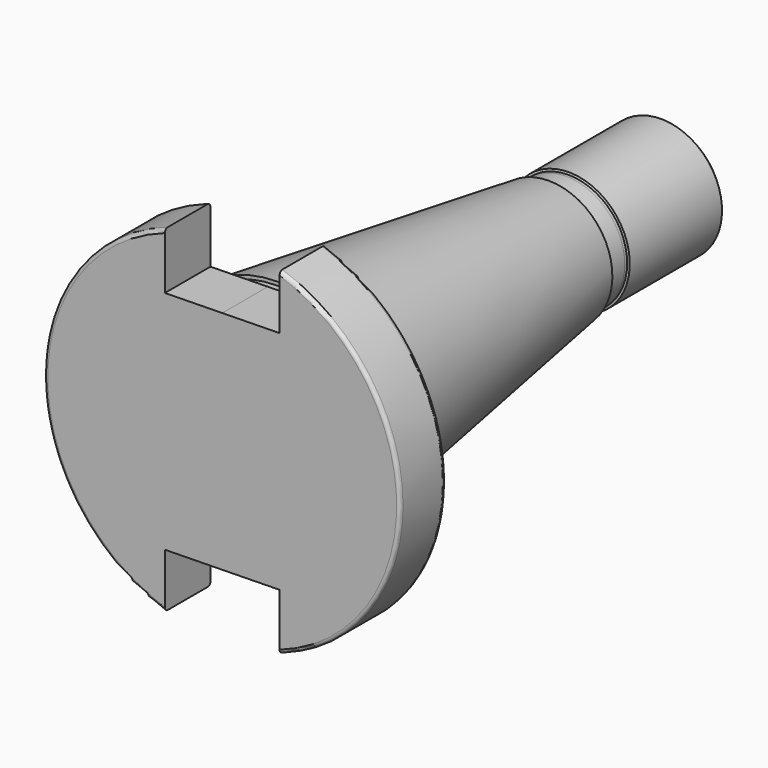
from build123d import *

# Parameters (mm, degrees)
F2_R             = 8.25
F3_DEPTH         = 3
F4_R             = 8.55
F5_DEPTH         = 17.2
F7_S5_R          = 8.25
F7_T6_DEPTH      = 14
F6_R             = 6.25
F8_DEPTH         = 4
F10_D            = 10.3
F10_DEPTH        = 25
F10_TIP          = 3.094432188
F11_R            = 0.5
F12_SIZE         = 0.5
F14_DEPTH        = 8
F14_COPIES_COUNT = 2


# Not quite as in the source:
# - a fillet or chamfer that OpenCascade refuses, or shapes differently, is made with other operations: its cross-section is extruded or revolved along the edge and cut away or added
# - a pattern or mirror of a feature is missing from the dataset's text; its kind, count and spacing are read off the source's solid


with BuildPart() as f1:
    # F0 (on Right) → F1 (revolve)
    with BuildSketch(Plane.YZ):
        Polygon((0, 25), (0, 0), (57.36, 0), (57.36, 8.9099957178), (9.6, 15.875), (9.6, 15.375), (8, 15.375), (8, 15.875), (8, 25), align=None)
    revolve(axis=Axis((0, 28.68, 0), (0, 1, 0)))

    # F2 (on face) → F3 (join)
    with BuildSketch(Plane(origin=(0, 57.36, 0), x_dir=(-1, 0, 0), z_dir=(0, 1, 0))):
        Circle(F2_R)
    extrude(amount=F3_DEPTH)

    # F4 (on face) → F5 (join)
    with BuildSketch(Plane(origin=(0, 60.36, 0), x_dir=(-1, 0, 0), z_dir=(0, 1, 0))):
        Circle(F4_R)
    extrude(amount=F5_DEPTH)

    # F7: chamfer of 0.5 x 1.8660254038 on 1 edges, made by hand


with BuildPart() as f7_tool2:
    # F7_s3 → F7_t4 (revolve)
    with BuildSketch(Plane.XY):
        Polygon((-8.55, 60.86), (-6.6839745962, 60.36), (-8.55, 60.36), align=None)
    revolve(axis=Axis((0, 60.36, 0), (0, 1, 0)))

    # F7_s5 → F7_t6 (cut, symmetric)
    with BuildSketch(Plane.XZ.offset(-60.6)):
        Circle(F7_S5_R)
    extrude(amount=F7_T6_DEPTH, both=True, mode=Mode.SUBTRACT)


with BuildPart() as f1_1:
    add(f1.part)

    # F7_t1: cut F7_tool2
    add(f7_tool2.part, mode=Mode.SUBTRACT)

    # F6 (on face) → F8 (cut)
    with BuildSketch(Plane(origin=(0, 77.56, 0), x_dir=(-1, 0, 0), z_dir=(0, 1, 0))):
        Circle(F6_R)
    extrude(amount=-F8_DEPTH, mode=Mode.SUBTRACT)

    # F10
    with Locations(Plane(origin=(0, 73.56, 0), x_dir=(-1, 0, 0), z_dir=(0, 1, 0))):
        with Locations((0, 0)):
            Hole(F10_D / 2, depth=F10_DEPTH)
            with Locations((0, 0, -(F10_DEPTH + F10_TIP / 2))):  # 118° drill point
                Cone(0, F10_D / 2, F10_TIP, mode=Mode.SUBTRACT)

    # F11
    f11_edges = [f1_1.edges().sort_by_distance(p)[0] for p in [
        (0, 8, -25),
        (0, 0, -25),
        (0, 4, 25),
    ]]
    fillet(f11_edges, radius=F11_R)

    # F12
    f12_edges = [f1_1.edges().sort_by_distance(p)[0] for p in [
        (8.55, 77.56, 0),
        (6.25, 77.56, 0),
        (5.15, 73.56, 0),
    ]]
    chamfer(f12_edges, length=F12_SIZE)

    # F13 (on face) → F14 (cut, through all)
    with BuildSketch(Plane.XZ):
        Polygon((-8.0518, 15.7346906059), (0, 15.8726696123), (8.0518, 16.0106486188), (8.0518, 25), (-8.0518, 25), align=None)
    f14 = extrude(amount=-F14_DEPTH, mode=Mode.SUBTRACT)

    # F14_copies: F14 ×2 about axis
    f14_copies_axis = Axis((0, 0, 0), (0, 1, 0))
    for i in range(1, F14_COPIES_COUNT):
        add(f14.rotate(f14_copies_axis, i * 360 / F14_COPIES_COUNT), mode=Mode.SUBTRACT)


solid = f1_1.part
